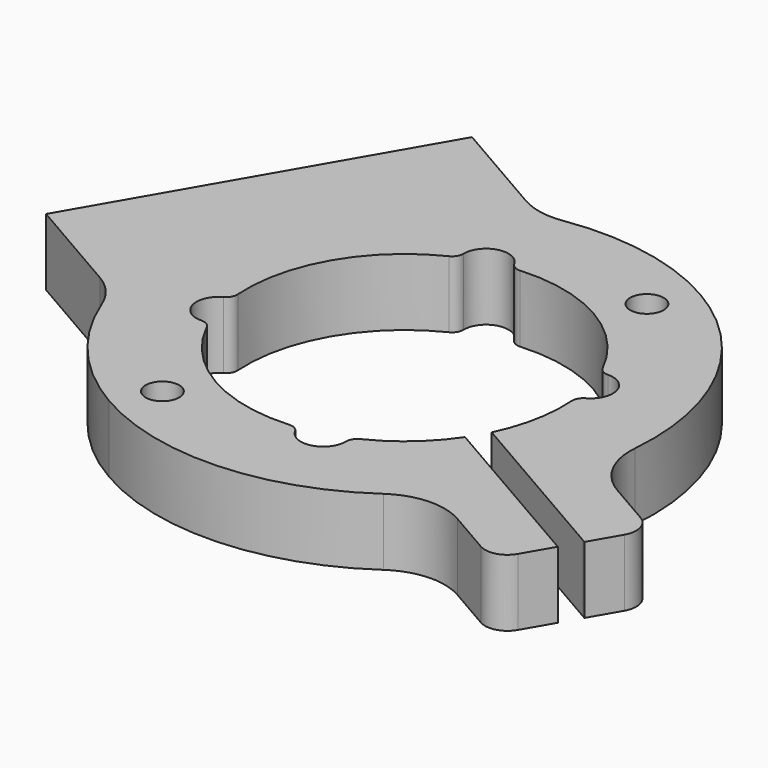
from build123d import *

# Parameters (mm, degrees)
F0_R     = 4.7625
F1_DEPTH = 19.05


# Not quite as in the source:
# - ends of sketch curves that miss each other by under 0.0002 mm in the source are joined


with BuildPart() as f1:
    # F0 (on Top) → F1 (new body)
    with BuildSketch(Plane.XY):
        with BuildLine():
            Line((-221.8857894, -106.4373771847), (-221.8857894, -88.1065191612))
            Line((-221.8857894, -88.1065191612), (-231.0306276, -82.826733))
            ThreePointArc((-231.0306276, -82.826733), (-238.3890078323, -75.1524401819), (-240.4883816501, -64.7297166236))
            ThreePointArc((-240.4883816501, -64.7297166236), (-248.2560543221, -26.1655958132), (-275.4820809487, 2.2293229893))
            ThreePointArc((-275.4820809487, 2.2293229893), (-297.7142880041, 10.461378966), (-321.4183295937, 10.8565858382))
            ThreePointArc((-321.4183295937, 10.8565858382), (-327.8248357317, 10.9634065797), (-333.8335467811, 13.1882885934))
            Line((-333.8335467811, 13.1882885934), (-362.314236, 29.6316146))
            Line((-362.314236, 29.6316146), (-413.114236, -58.3565508))
            Line((-413.114236, -58.3565508), (-384.6335462, -74.7999012))
            ThreePointArc((-384.6335462, -74.7999012), (-379.7023894379, -78.8911519852), (-376.4066376642, -84.3859370356))
            ThreePointArc((-376.4066376642, -84.3859370356), (-364.2123588019, -104.7166445735), (-345.9670808498, -119.8542782393))
            ThreePointArc((-345.9670808498, -119.8542782393), (-307.7633473097, -129.2352495129), (-270.4820087562, -116.6801838382))
            ThreePointArc((-270.4820087562, -116.6801838382), (-260.4059713642, -113.286900565), (-250.0806270189, -115.8222971934))
            Line((-250.0806270189, -115.8222971934), (-237.760637, -122.9352634))
            ThreePointArc((-237.760637, -122.9352634), (-232.9421342351, -123.569614107), (-229.0863779145, -120.6109894599))
            Line((-229.0863779145, -120.6109894599), (-224.3238846, -112.362107))
            Line((-224.3238846, -112.362107), (-273.3642488, -84.0486254))
            ThreePointArc((-273.3642488, -84.0486254), (-281.1433177605, -92.8360964437), (-290.9268252362, -99.3181139076))
            ThreePointArc((-290.9268252362, -99.3181139076), (-292.2425670349, -100.5162816603), (-292.7069827203, -102.2341617784))
            ThreePointArc((-292.7069827203, -102.2341617784), (-297.4122125633, -108.4948669165), (-304.6174116153, -105.4255515302))
            ThreePointArc((-304.6174116153, -105.4255515302), (-305.8785439427, -104.1700351993), (-307.6170882048, -103.7902477201))
            ThreePointArc((-307.6170882048, -103.7902477201), (-333.2670739258, -97.8572369807), (-351.2302185284, -78.6102104616))
            ThreePointArc((-351.2302185284, -78.6102104616), (-352.4283762603, -77.2944637651), (-354.1462563784, -76.8300480797))
            ThreePointArc((-354.1462563784, -76.8300480797), (-360.4069615165, -72.1248182367), (-357.3376461302, -64.9196191847))
            ThreePointArc((-357.3376461302, -64.9196191847), (-356.0821208015, -63.6584957522), (-355.7023440666, -61.9199427159))
            ThreePointArc((-355.7023440666, -61.9199427159), (-349.7693252458, -36.2699713018), (-330.5223050616, -18.3068376716))
            ThreePointArc((-330.5223050616, -18.3068376716), (-329.2065612709, -17.1086592996), (-328.7421426797, -15.3907744216))
            ThreePointArc((-328.7421426797, -15.3907744216), (-324.0369128367, -9.1300692835), (-316.8317137847, -12.1993846698))
            ThreePointArc((-316.8317137847, -12.1993846698), (-315.5705903522, -13.4549099985), (-313.8320373159, -13.8346867334))
            ThreePointArc((-313.8320373159, -13.8346867334), (-288.1820750251, -19.7677256868), (-270.2189422924, -39.0147306362))
            ThreePointArc((-270.2189422924, -39.0147306362), (-269.0207538996, -40.3304695291), (-267.3028690216, -40.7948881203))
            ThreePointArc((-267.3028690216, -40.7948881203), (-261.0421638835, -45.5001179633), (-264.1114792698, -52.7053170153))
            ThreePointArc((-264.1114792698, -52.7053170153), (-265.3669956007, -53.9664493427), (-265.7467830799, -55.7049936048))
            ThreePointArc((-265.7467830799, -55.7049936048), (-266.4686255378, -67.4187649457), (-270.1892527015, -78.5493711003))
            Line((-270.1892527015, -78.5493711003), (-221.8857894, -106.4373771847))
        make_face()
        with Locations((-339.6170754, -108.8557386)):
            Circle(F0_R, mode=Mode.SUBTRACT)
        with Locations((-281.8320754, -8.7691976)):
            Circle(F0_R, mode=Mode.SUBTRACT)
        with BuildLine():
            Line((-218.710637, -89.9396982), (-221.8857894, -88.1065191612))
            Line((-221.8857894, -88.1065191612), (-221.8857894, -106.4373771847))
            Line((-221.8857894, -106.4373771847), (-221.1488846, -106.8628292))
            Line((-221.1488846, -106.8628292), (-216.3863846, -98.6139506))
            ThreePointArc((-216.3863846, -98.6139506), (-215.7520068495, -93.7954539688), (-218.710637, -89.9396982))
        make_face()
    extrude(amount=F1_DEPTH)


solid = f1.part
